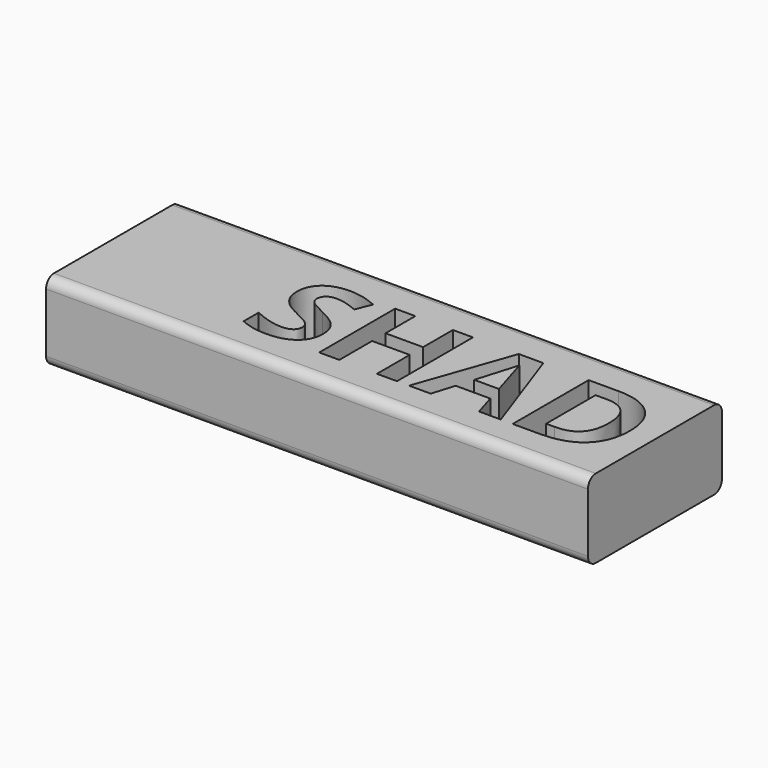
from build123d import *

# Parameters (mm, degrees)
F0_W         = 17
F0_H         = 8
F1_DEPTH     = 55
F2_R         = 1
F3_W         = 12.4
F3_H         = 5
F4_DEPTH     = 14
F5_ANGLE     = 90
F6_TEXT_SIZE = 13.4957776431
F7_DEPTH     = 5


# Not quite as in the source:
# - Text() gives the source's letters only with a copy of the font that has no kerning and outlines rounded to 1/6400 em; it was checked with that copy


with BuildPart() as f1:
    # F0 (on Front) → F1 (new body)
    with BuildSketch(Plane.XZ):
        Rectangle(F0_W, F0_H)
    extrude(amount=F1_DEPTH)

    # F2
    f2_edges = [f1.edges().sort_by_distance(p)[0] for p in [
        (8.5, -27.5, 4),
        (-8.5, -27.5, 4),
        (8.5, -27.5, -4),
        (-8.5, -27.5, -4),
    ]]
    fillet(f2_edges, radius=F2_R)

    # F3 (on face) → F4 (cut)
    with BuildSketch(Plane(origin=(0, 0, 0), x_dir=(-1, 0, 0), z_dir=(0, 1, 0))):
        Rectangle(F3_W, F3_H)
    extrude(amount=-F4_DEPTH, mode=Mode.SUBTRACT)


with BuildPart() as f1_1:
    # F5: moved
    add(f1.part.rotate(Axis((8.5, 0, 0), (0, 0, 1)), F5_ANGLE))

    # F6 (on face) → F7 (cut)
    with BuildSketch(Plane.XY.offset(4)):
        with Locations((24.7637610883, -13.4812160395)):
            Text('SHAD', F6_TEXT_SIZE, font='Open Sans', font_style=FontStyle.BOLD, text_align=(TextAlign.LEFT, TextAlign.BOTTOM))
    extrude(amount=-F7_DEPTH, mode=Mode.SUBTRACT)


solid = f1_1.part
